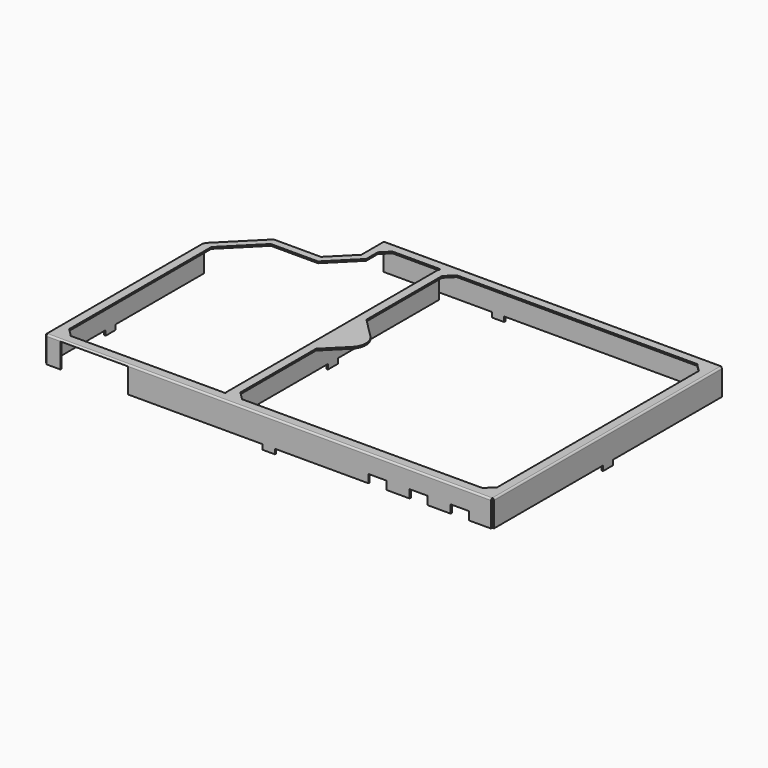
from build123d import *

# Parameters (mm, degrees)
F0_W     = 0.2
F0_H     = 1.5
F0_H_2   = 8.8
F1_DEPTH = 3
F0_W_2   = 1.7
F0_H_3   = 0.2
F0_W_3   = 16.35
F0_W_4   = 1.5
F0_W_5   = 11.35
F0_W_6   = 2.199999
F0_W_7   = 2.800001
F0_W_8   = 2.700001
F0_H_4   = 15.349983
F0_H_5   = 15.349984
F0_H_6   = 16.549983
F0_H_7   = 16.549984
F0_W_9   = 26.25
F0_W_10  = 13.149958
F2_START = 3
F2_DEPTH = 0.2
F3_DEPTH = 1
F4_DEPTH = 0.6
F5_R     = 0.1999


# Not quite as in the source:
# - a fillet or chamfer is up to 0.001 mm smaller than in the source, because OpenCascade refuses the exact size
# - ends of sketch curves that miss each other by under 0.0002 mm in the source are joined


with BuildPart() as f1:
    # F0 (on Top) → F1 (new body)
    with BuildSketch(Plane.XY):
        with Locations((-26.40002, -7.749967)):
            Rectangle(F0_W, F0_H)
        Polygon((-26.30002, 6.400033), (-26.50002, 6.400037), (-26.50002, -6.999967), (-26.30002, -6.999967), align=None)
        with Locations((-26.40002, -12.899967)):
            Rectangle(F0_W, F0_H_2)
    extrude(amount=F1_DEPTH)

    # F0 (on Top) → F4, piece 3 (join)
    with BuildSketch(Plane.XY):
        with Locations((-26.40002, -7.749967)):
            Rectangle(F0_W, F0_H)
    extrude(amount=-F4_DEPTH)


with BuildPart() as f1b:
    # F0 (on Top) → F1, piece 2 (new body)
    with BuildSketch(Plane.XY):
        with Locations((-25.45002, -17.399967)):
            Rectangle(F0_W_2, F0_H_3)
    extrude(amount=F1_DEPTH)


with BuildPart() as f1c:
    # F0 (on Top) → F1, piece 3 (new body)
    with BuildSketch(Plane.XY):
        with Locations((-8.22502, -17.399967)):
            Rectangle(F0_W_3, F0_H_3)
        with Locations((0.69998, -17.399967)):
            Rectangle(F0_W_4, F0_H_3)
        with Locations((7.12498, -17.399967)):
            Rectangle(F0_W_5, F0_H_3)
        with Locations((13.8999795, -17.399967)):
            Rectangle(F0_W_6, F0_H_3)
        with Locations((16.3999795, -17.399967)):
            Rectangle(F0_W_7, F0_H_3)
        with Locations((18.8999795, -17.399967)):
            Rectangle(F0_W_6, F0_H_3)
        with Locations((21.3999795, -17.399967)):
            Rectangle(F0_W_7, F0_H_3)
        with Locations((23.8999795, -17.399967)):
            Rectangle(F0_W_6, F0_H_3)
        with Locations((26.3499795, -17.399967)):
            Rectangle(F0_W_8, F0_H_3)
    extrude(amount=F1_DEPTH)

    # F0 (on Top) → F3 (cut)
    with BuildSketch(Plane.XY):
        with Locations((13.8999795, -17.399967)):
            Rectangle(F0_W_6, F0_H_3)
        with Locations((18.8999795, -17.399967)):
            Rectangle(F0_W_6, F0_H_3)
        with Locations((23.8999795, -17.399967)):
            Rectangle(F0_W_6, F0_H_3)
    extrude(amount=F3_DEPTH, mode=Mode.SUBTRACT)

    # F0 (on Top) → F4 (join)
    with BuildSketch(Plane.XY):
        with Locations((0.69998, -17.399967)):
            Rectangle(F0_W_4, F0_H_3)
    extrude(amount=-F4_DEPTH)


with BuildPart() as f1d:
    # F0 (on Top) → F1, piece 4 (new body)
    with BuildSketch(Plane.XY):
        with Locations((-5.60002, -8.4249755)):
            Rectangle(F0_W, F0_H_4)
        with Locations((-5.60002, 1.6e-05)):
            Rectangle(F0_W, F0_H)
        with Locations((-5.60002, 8.425008)):
            Rectangle(F0_W, F0_H_5)
    extrude(amount=F1_DEPTH)

    # F0 (on Top) → F4, piece 2 (join)
    with BuildSketch(Plane.XY):
        with Locations((-5.60002, 1.6e-05)):
            Rectangle(F0_W, F0_H)
    extrude(amount=-F4_DEPTH)


with BuildPart() as f1e:
    # F0 (on Top) → F1, piece 5 (new body)
    with BuildSketch(Plane.XY):
        with Locations((27.79998, -9.0249755)):
            Rectangle(F0_W, F0_H_6)
        with Locations((27.79998, 1.6e-05)):
            Rectangle(F0_W, F0_H)
        with Locations((27.79998, 9.025008)):
            Rectangle(F0_W, F0_H_7)
    extrude(amount=F1_DEPTH)

    # F0 (on Top) → F4, piece 5 (join)
    with BuildSketch(Plane.XY):
        with Locations((27.79998, 1.6e-05)):
            Rectangle(F0_W, F0_H)
    extrude(amount=-F4_DEPTH)


with BuildPart() as f1f:
    # F0 (on Top) → F1, piece 6 (new body)
    with BuildSketch(Plane.XY):
        with Locations((14.57498, 17.4)):
            Rectangle(F0_W_9, F0_H_3)
        with Locations((0.69998, 17.4)):
            Rectangle(F0_W_4, F0_H_3)
        with Locations((-6.624999, 17.4)):
            Rectangle(F0_W_10, F0_H_3)
    extrude(amount=F1_DEPTH)

    # F0 (on Top) → F4, piece 4 (join)
    with BuildSketch(Plane.XY):
        with Locations((0.69998, 17.4)):
            Rectangle(F0_W_4, F0_H_3)
    extrude(amount=-F4_DEPTH)


with BuildPart() as f2:
    # F0 (on Top) → F2 (new body)
    with BuildSketch(Plane.XY.offset(F2_START)):
        Polygon((-26.30002, 6.500037), (-26.30002, 6.400033), (-26.30002, -6.999967), (-26.30002, -8.499967), (-26.30002, -17.299967), (-24.60002, -17.299967), (-24.60002, -17.499967), (-16.40002, -17.499967), (-16.40002, -17.299967), (-0.05002, -17.299967), (1.44998, -17.299967), (12.79998, -17.299967), (14.999979, -17.299967), (17.79998, -17.299967), (19.999979, -17.299967), (22.79998, -17.299967), (24.999979, -17.299967), (27.69998, -17.299967), (27.69998, -0.749984), (27.69998, 0.750016), (27.69998, 17.3), (1.44998, 17.3), (-0.05002, 17.3), (-13.199978, 17.3), (-13.199978, 13.925762), (-15.925703, 11.200037), (-21.658599, 11.200037), (-26.30002, 6.558616), align=None)
        Polygon((-25.30002, -15.299967), (-25.30002, 6.28582), (-21.285807, 10.300037), (-15.55291, 10.300037), (-12.299978, 13.55297), (-12.299978, 15.3), (-11.299978, 16.3), (-5.50002, 16.3), (-5.50002, 16.1), (-5.50002, 0.750016), (-5.50002, -0.749984), (-5.50002, -16.099967), (-5.50002, -16.299967), (-24.30002, -16.299967), align=None, mode=Mode.SUBTRACT)
        with BuildLine():
            Line((25.69998, 16.3), (26.69998, 15.3))
            Line((26.69998, 15.3), (26.69998, -15.299967))
            Line((26.69998, -15.299967), (25.69998, -16.299967))
            Line((25.69998, -16.299967), (-3.50002, -16.299967))
            Line((-3.50002, -16.299967), (-4.50002, -15.299967))
            Line((-4.50002, -15.299967), (-4.50002, -3.828411))
            Line((-4.50002, -3.828411), (-2.085807, -1.414197))
            ThreePointArc((-2.085807, -1.414197), (-1.50002, 1.63536e-05), (-2.0858069376, 1.4142300624))
            Line((-2.0858069376, 1.4142300624), (-4.500051, 3.828581))
            Line((-4.500051, 3.828581), (-4.50002, 15.3))
            Line((-4.50002, 15.3), (-3.50002, 16.3))
            Line((-3.50002, 16.3), (25.69998, 16.3))
        make_face(mode=Mode.SUBTRACT)
        with Locations((-25.45002, -17.399967)):
            Rectangle(F0_W_2, F0_H_3)
        with Locations((-26.40002, -12.899967)):
            Rectangle(F0_W, F0_H_2)
        with Locations((-26.40002, -7.749967)):
            Rectangle(F0_W, F0_H)
        Polygon((-26.30002, 6.400033), (-26.50002, 6.400037), (-26.50002, -6.999967), (-26.30002, -6.999967), align=None)
        with Locations((-6.624999, 17.4)):
            Rectangle(F0_W_10, F0_H_3)
        with Locations((-5.60002, 8.425008)):
            Rectangle(F0_W, F0_H_5)
        with Locations((-5.60002, 1.6e-05)):
            Rectangle(F0_W, F0_H)
        with Locations((-5.60002, -8.4249755)):
            Rectangle(F0_W, F0_H_4)
        with Locations((-8.22502, -17.399967)):
            Rectangle(F0_W_3, F0_H_3)
        with Locations((0.69998, -17.399967)):
            Rectangle(F0_W_4, F0_H_3)
        with Locations((7.12498, -17.399967)):
            Rectangle(F0_W_5, F0_H_3)
        with Locations((13.8999795, -17.399967)):
            Rectangle(F0_W_6, F0_H_3)
        with Locations((16.3999795, -17.399967)):
            Rectangle(F0_W_7, F0_H_3)
        with Locations((18.8999795, -17.399967)):
            Rectangle(F0_W_6, F0_H_3)
        with Locations((21.3999795, -17.399967)):
            Rectangle(F0_W_7, F0_H_3)
        with Locations((23.8999795, -17.399967)):
            Rectangle(F0_W_6, F0_H_3)
        with Locations((26.3499795, -17.399967)):
            Rectangle(F0_W_8, F0_H_3)
        with Locations((27.79998, -9.0249755)):
            Rectangle(F0_W, F0_H_6)
        with Locations((27.79998, 1.6e-05)):
            Rectangle(F0_W, F0_H)
        with Locations((27.79998, 9.025008)):
            Rectangle(F0_W, F0_H_7)
        with Locations((14.57498, 17.4)):
            Rectangle(F0_W_9, F0_H_3)
        with Locations((0.69998, 17.4)):
            Rectangle(F0_W_4, F0_H_3)
    extrude(amount=F2_DEPTH)

    # F5 (radius 0.2 in the source; OpenCascade refuses exactly that, so slightly less here)
    f5_edges = [f2.edges().sort_by_distance(p)[0] for p in [
        (0.69998, -17.499967, 3.2),
        (27.89998, 1.7e-05, 3.2),
        (7.250001, 17.5, 3.2),
        (-26.50002, -5.449965, 3.2),
        (-5.70002, 1.7e-05, 3.2),
    ]]
    fillet(f5_edges, radius=F5_R)


solid = Compound([f1.part, f1b.part, f1c.part, f1d.part, f1e.part, f1f.part, f2.part])
